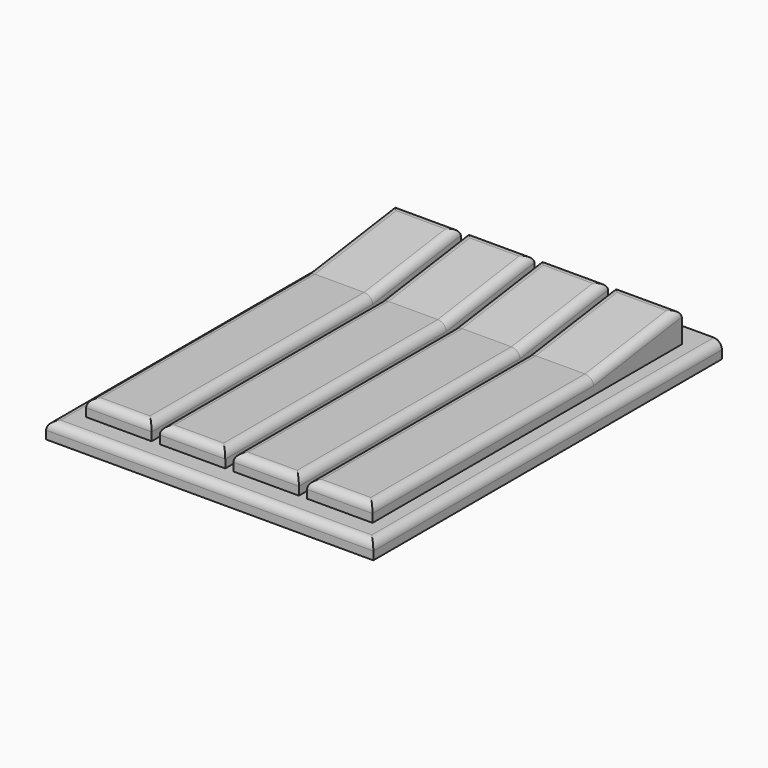
from build123d import *

# Parameters (mm, degrees)
F0_W         = 10.16
F0_H         = 17.20733324
F1_DEPTH     = 7.62
F0_H_2       = 42.8125401959
F2_DEPTH     = 5.08
F0_W_2       = 50.8
F0_H_3       = 67.63987211
F3_DEPTH     = 2.54
F4_T4_DEPTH  = 102.5816286105
F4_T9_DEPTH  = 102.5816286105
F4_T14_DEPTH = 102.5816286105
F4_T19_DEPTH = 102.5816286105
F5_R         = 1.27
F6_R         = 1.27


# Not quite as in the source:
# - a fillet or chamfer that OpenCascade refuses, or shapes differently, is made with other operations: its cross-section is extruded or revolved along the edge and cut away or added
# - two fillets or chamfers of one size are made in one step
# - ends of sketch curves that miss each other by under 0.0002 mm in the source are joined


with BuildPart() as f1:
    # F0 (on Top) → F1 (new body)
    with BuildSketch(Plane.XY):
        with Locations((-17.1449951105, 21.4062702746)):
            Rectangle(F0_W, F0_H)
    extrude(amount=F1_DEPTH)

    # F0 (on Top) → F2 (join)
    with BuildSketch(Plane.XY):
        with Locations((-17.1449951105, 21.4062702746)):
            Rectangle(F0_W, F0_H)
        with Locations((-17.1449951105, -8.6036664434)):
            Rectangle(F0_W, F0_H_2)
    extrude(amount=F2_DEPTH)



with BuildPart() as f1b:
    # F0 (on Top) → F1, piece 2 (new body)
    with BuildSketch(Plane.XY):
        with Locations((-5.7149951105, 21.4062702746)):
            Rectangle(F0_W, F0_H)
    extrude(amount=F1_DEPTH)

    # F0 (on Top) → F2, piece 2 (join)
    with BuildSketch(Plane.XY):
        with Locations((-5.7149951105, -8.6036664434)):
            Rectangle(F0_W, F0_H_2)
        with Locations((-5.7149951105, 21.4062702746)):
            Rectangle(F0_W, F0_H)
    extrude(amount=F2_DEPTH)


with BuildPart() as f1c:
    # F0 (on Top) → F1, piece 3 (new body)
    with BuildSketch(Plane.XY):
        with Locations((5.7150048895, 21.4062702746)):
            Rectangle(F0_W, F0_H)
    extrude(amount=F1_DEPTH)

    # F0 (on Top) → F2, piece 3 (join)
    with BuildSketch(Plane.XY):
        with Locations((5.7150048895, -8.6036664434)):
            Rectangle(F0_W, F0_H_2)
        with Locations((5.7150048895, 21.4062702746)):
            Rectangle(F0_W, F0_H)
    extrude(amount=F2_DEPTH)


with BuildPart() as f1d:
    # F0 (on Top) → F1, piece 4 (new body)
    with BuildSketch(Plane.XY):
        with Locations((17.1450048895, 21.4062702746)):
            Rectangle(F0_W, F0_H)
    extrude(amount=F1_DEPTH)

    # F0 (on Top) → F2, piece 4 (join)
    with BuildSketch(Plane.XY):
        with Locations((17.1450048895, -8.6036664434)):
            Rectangle(F0_W, F0_H_2)
        with Locations((17.1450048895, 21.4062702746)):
            Rectangle(F0_W, F0_H)
    extrude(amount=F2_DEPTH)


with BuildPart() as f1_1:
    add(f1.part)

    add(f1b.part)  # F3 merges F1b

    add(f1c.part)  # F3 merges F1c

    add(f1d.part)  # F3 merges F1d
    # F0 (on Top) → F3 (join)
    with BuildSketch(Plane.XY):
        with Locations((0, -1.609e-07)):
            Rectangle(F0_W_2, F0_H_3)
        Polygon((-22.2249951105, 30.0099368946), (-12.0649951105, 30.0099368946), (-12.0649951105, 12.8026036546), (-12.0649951105, -30.0099365413), (-22.2249951105, -30.0099365413), (-22.2249951105, 12.8026036546), align=None, mode=Mode.SUBTRACT)
        Polygon((-10.7949951105, -30.0099365413), (-10.7949951105, 12.8026036546), (-10.7949951105, 30.0099368946), (-0.6349951105, 30.0099368946), (-0.6349951105, 12.8026036546), (-0.6349951105, -30.0099365413), align=None, mode=Mode.SUBTRACT)
        Polygon((0.6350048895, -30.0099365413), (0.6350048895, 12.8026036546), (0.6350048895, 30.0099368946), (10.7950048895, 30.0099368946), (10.7950048895, 12.8026036546), (10.7950048895, -30.0099365413), align=None, mode=Mode.SUBTRACT)
        Polygon((12.0650048895, -30.0099365413), (12.0650048895, 12.8026036546), (12.0650048895, 30.0099368946), (22.2250048895, 30.0099368946), (22.2250048895, 12.8026036546), (22.2250048895, -30.0099365413), align=None, mode=Mode.SUBTRACT)
    extrude(amount=F3_DEPTH)

    # F4: chamfer of 17.78 x 2.54 on 4 edges, made by hand


with BuildPart() as f4_tool2:
    # F4_s3 → F4_t4 (new body)
    with BuildSketch(Plane.YZ.offset(-68.4358094158)):
        Polygon((30.5826036546, 7.62), (12.8026036546, 5.08), (12.8026036546, 7.62), align=None)
    extrude(amount=F4_T4_DEPTH)

    split(bisect_by=Plane.XY.offset(5.08), keep=Keep.TOP)


with BuildPart() as f1_2:
    add(f1_1.part)

    # F4_t1: cut F4_tool2
    add(f4_tool2.part, mode=Mode.SUBTRACT)


with BuildPart() as f4_tool7:
    # F4_s8 → F4_t9 (new body)
    with BuildSketch(Plane.YZ.offset(-57.0058094158)):
        Polygon((12.8026036546, 5.08), (30.5826036546, 7.62), (12.8026036546, 7.62), align=None)
    extrude(amount=F4_T9_DEPTH)

    split(bisect_by=Plane.XY.offset(5.08), keep=Keep.TOP)


with BuildPart() as f1_3:
    add(f1_2.part)

    # F4_t6: cut F4_tool7
    add(f4_tool7.part, mode=Mode.SUBTRACT)


with BuildPart() as f4_tool12:
    # F4_s13 → F4_t14 (new body)
    with BuildSketch(Plane.YZ.offset(-45.5758094158)):
        Polygon((12.8026036546, 5.08), (30.5826036546, 7.62), (12.8026036546, 7.62), align=None)
    extrude(amount=F4_T14_DEPTH)

    split(bisect_by=Plane.XY.offset(5.08), keep=Keep.TOP)


with BuildPart() as f1_4:
    add(f1_3.part)

    # F4_t11: cut F4_tool12
    add(f4_tool12.part, mode=Mode.SUBTRACT)


with BuildPart() as f4_tool17:
    # F4_s18 → F4_t19 (new body)
    with BuildSketch(Plane.YZ.offset(-34.1458094158)):
        Polygon((12.8026036546, 5.08), (30.5826036546, 7.62), (12.8026036546, 7.62), align=None)
    extrude(amount=F4_T19_DEPTH)

    split(bisect_by=Plane.XY.offset(5.08), keep=Keep.TOP)


with BuildPart() as f1_5:
    add(f1_4.part)

    # F4_t16: cut F4_tool17
    add(f4_tool17.part, mode=Mode.SUBTRACT)

    # F5
    f5_edges = [f1_5.edges().sort_by_distance(p)[0] for p in [
        (0, -33.819936, 2.54),
        (-25.4, 0, 2.54),
        (25.4, 0, 2.54),
    ]]
    fillet(f5_edges, radius=F5_R)

    # F6
    f6_edges = [f1_5.edges().sort_by_distance(p)[0] for p in [
        (-12.064995, -8.603666, 5.08),
        (-17.144995, -30.009937, 5.08),
        (-22.224995, -8.603666, 5.08),
        (-5.714995, -30.009937, 5.08),
        (-10.794995, -8.603666, 5.08),
        (-0.634995, -8.603666, 5.08),
        (0.635005, -8.603666, 5.08),
        (10.795005, -8.603666, 5.08),
        (5.715005, -30.009937, 5.08),
        (17.145005, -30.009937, 5.08),
        (12.065005, -8.603666, 5.08),
        (22.225005, -8.603666, 5.08),
        (-17.144995, 30.009937, 7.53819),
        (-12.064995, 21.40627, 6.309095),
        (-22.224995, 21.40627, 6.309095),
        (-10.794995, 21.40627, 6.309095),
        (-5.714995, 30.009937, 7.53819),
        (-0.634995, 21.40627, 6.309095),
        (0.635005, 21.40627, 6.309095),
        (5.715005, 30.009937, 7.53819),
        (10.795005, 21.40627, 6.309095),
        (12.065005, 21.40627, 6.309095),
        (17.145005, 30.009937, 7.53819),
        (22.225005, 21.40627, 6.309095),
    ]]
    fillet(f6_edges, radius=F6_R)


solid = f1_5.part
